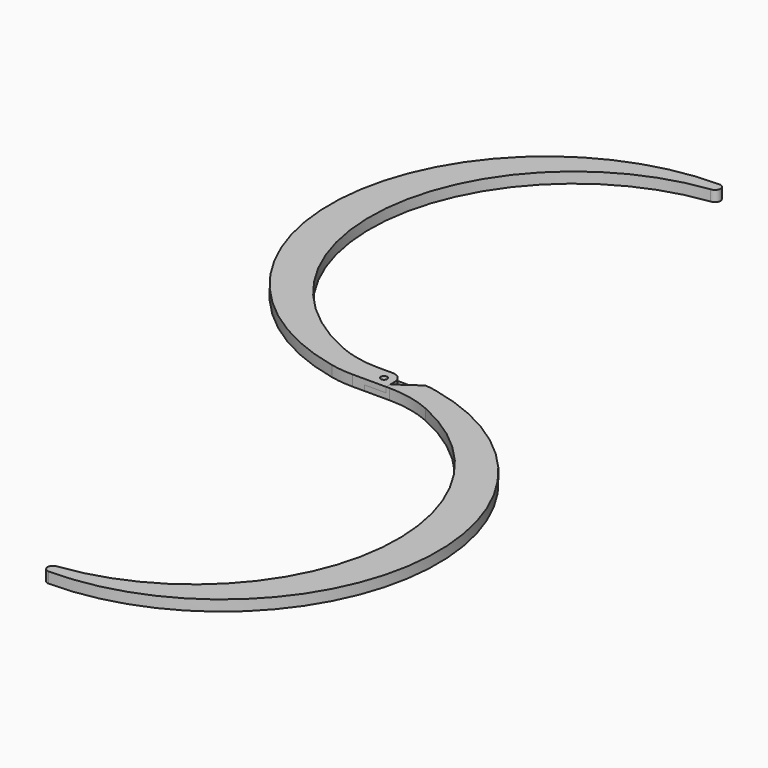
from build123d import *

# Parameters (mm, degrees)
F1_DEPTH  = 10
F2_R      = 3
F3_DEPTH  = 25
F6_DEPTH  = 5
F10_DEPTH = 5
F12_DEPTH = 5
F13_DEPTH = 5
F15_DEPTH = 5
F16_DEPTH = 5


with BuildPart() as f1:
    # F0 (on Top) → F1 (new body)
    with BuildSketch(Plane.XY):
        with BuildLine():
            ThreePointArc((0, 380), (5, 385), (0, 390))
            ThreePointArc((0, 390), (-200.0031288383, 210.088535299), (-42.1904132607, -7.7750309023))
            ThreePointArc((-42.1904132607, -7.7750309023), (-31.7606417446, -9.4422020327), (-21.2132034356, -10))
            Line((-21.2132034356, -10), (0, -10))
            Line((0, -10), (12.9417308956, -10))
            ThreePointArc((12.9417308956, -10), (33.5719267784, -12.1511624094), (53.3145446236, -18.5120996432))
            ThreePointArc((53.3145446236, -18.5120996432), (164.29346462, -219.555514643), (0, -380))
            ThreePointArc((0, -380), (-5, -385), (0, -390))
            ThreePointArc((0, -390), (200.0031288383, -210.088535299), (42.1904132607, 7.7750309023))
            ThreePointArc((42.1904132607, 7.7750309023), (31.7606417446, 9.4422020327), (21.2132034356, 10))
            Line((21.2132034356, 10), (0, 10))
            Line((0, 10), (-12.9417308956, 10))
            ThreePointArc((-12.9417308956, 10), (-33.5719267784, 12.1511624094), (-53.3145446236, 18.5120996432))
            ThreePointArc((-53.3145446236, 18.5120996432), (-164.29346462, 219.555514643), (0, 380))
        make_face()
    extrude(amount=F1_DEPTH)

    # F2 (on face) → F3 (cut)
    with BuildSketch(Plane.XY.offset(10)):
        Circle(F2_R)
        with BuildLine():
            ThreePointArc((0, 10), (10, 0), (0, -10))
            Line((0, -10), (12.9417308956, -10))
            ThreePointArc((12.9417308956, -10), (33.5719267784, -12.1511624094), (53.3145446236, -18.5120996432))
            ThreePointArc((53.3145446236, -18.5120996432), (164.29346462, -219.555514643), (0, -380))
            ThreePointArc((0, -380), (-5, -385), (0, -390))
            ThreePointArc((0, -390), (200.0031288383, -210.088535299), (42.1904132607, 7.7750309023))
            ThreePointArc((42.1904132607, 7.7750309023), (31.7606417446, 9.4422020327), (21.2132034356, 10))
            Line((21.2132034356, 10), (0, 10))
        make_face()
    extrude(amount=-F3_DEPTH, mode=Mode.SUBTRACT)


with BuildPart() as f4_1:
    # F4: instance of F1
    add(f1.part.mirror(Plane.YZ))


with BuildPart() as f1_1:
    add(f1.part)

    # F5 (on face) → F6 (cut)
    with BuildSketch(Plane(origin=(0, 0, 0), x_dir=(1, 0, 0), z_dir=(0, 0, -1))):
        with BuildLine():
            ThreePointArc((0, -10), (7.0710678119, -7.0710678119), (10, 0))
            ThreePointArc((10, 0), (4.6174861324, 8.8701083318), (-5.7357643635, 8.1915204429))
            ThreePointArc((-5.7357643635, 8.1915204429), (-9.5371695075, -3.007057995), (0, -10))
        make_face()
        with BuildLine():
            ThreePointArc((0, -10), (-9.5371695075, -3.007057995), (-5.7357643635, 8.1915204429))
            Line((-5.7357643635, 8.1915204429), (-35.3465892462, -12.5422023525))
            ThreePointArc((-35.3465892462, -12.5422023525), (-24.2160431863, -10.6375831495), (-12.9417308956, -10))
            Line((-12.9417308956, -10), (0, -10))
        make_face()
    extrude(amount=-F6_DEPTH, mode=Mode.SUBTRACT)

    # F11 (on face) → F13 (cut)
    with BuildSketch(Plane(origin=(0, 0, 0), x_dir=(1, 0, 0), z_dir=(0, 0, -1))):
        with BuildLine():
            ThreePointArc((-10, 0), (-7.0710678119, 7.0710678119), (0, 10))
            Line((0, 10), (-10, 10))
            Line((-10, 10), (-10, 0))
        make_face()
    extrude(amount=-F13_DEPTH, mode=Mode.SUBTRACT)

    # F14 (on face) → F15 (join)
    with BuildSketch(Plane.XY.offset(10)):
        with BuildLine():
            ThreePointArc((10, 0), (7.0710678119, -7.0710678119), (0, -10))
            Line((0, -10), (10, -10))
            Line((10, -10), (10, 0))
        make_face()
    extrude(amount=-F15_DEPTH)


with BuildPart() as f7_1:
    # F7: instance of F4_1
    add(f4_1.part.mirror(Plane.XZ))

    # F9 (on face) → F10 (cut)
    with BuildSketch(Plane.XY.offset(10)):
        with BuildLine():
            ThreePointArc((5.7357643635, -8.1915204429), (8.8701083318, -4.6174861324), (10, 0))
            ThreePointArc((10, 0), (7.0710678119, 7.0710678119), (0, 10))
            ThreePointArc((0, 10), (-9.5371695075, -3.007057995), (5.7357643635, -8.1915204429))
        make_face()
        with BuildLine():
            ThreePointArc((0, 10), (7.0710678119, 7.0710678119), (10, 0))
            ThreePointArc((10, 0), (8.8701083318, -4.6174861324), (5.7357643635, -8.1915204429))
            Line((5.7357643635, -8.1915204429), (31.0266100505, 9.5173203549))
            ThreePointArc((31.0266100505, 9.5173203549), (26.1258383963, 9.8792571946), (21.2132034356, 10))
            Line((21.2132034356, 10), (0, 10))
        make_face()
    extrude(amount=-F10_DEPTH, mode=Mode.SUBTRACT)

    # F11 (on face) → F12 (join)
    with BuildSketch(Plane(origin=(0, 0, 0), x_dir=(1, 0, 0), z_dir=(0, 0, -1))):
        with BuildLine():
            ThreePointArc((-10, 0), (-7.0710678119, 7.0710678119), (0, 10))
            Line((0, 10), (-10, 10))
            Line((-10, 10), (-10, 0))
        make_face()
    extrude(amount=-F12_DEPTH)

    # F14 (on face) → F16 (cut)
    with BuildSketch(Plane.XY.offset(10)):
        with BuildLine():
            ThreePointArc((10, 0), (7.0710678119, -7.0710678119), (0, -10))
            Line((0, -10), (10, -10))
            Line((10, -10), (10, 0))
        make_face()
    extrude(amount=-F16_DEPTH, mode=Mode.SUBTRACT)


solid = Compound([f1_1.part, f7_1.part])
